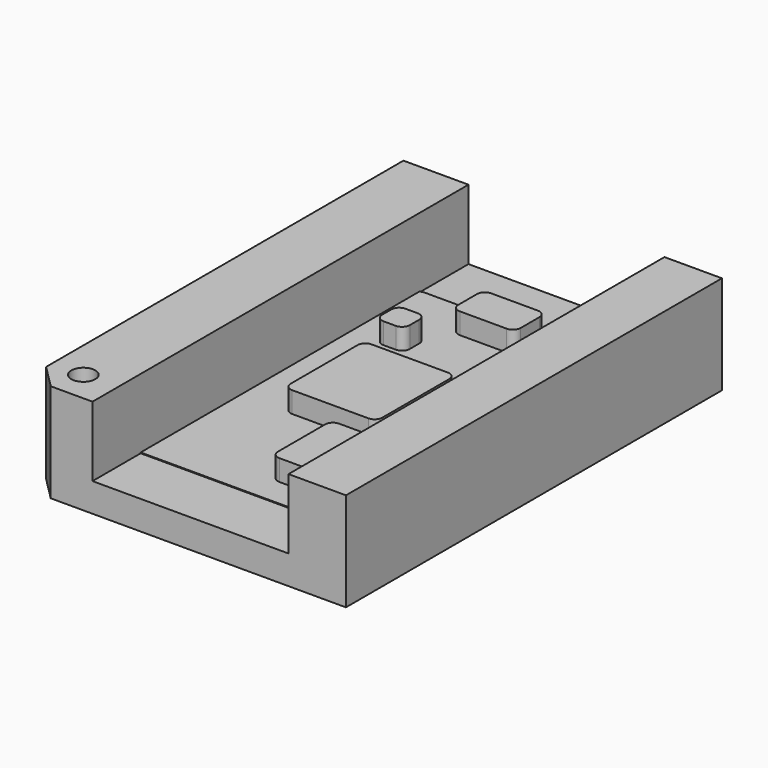
from build123d import *

# Parameters (mm, degrees)
F0_W      = 41
F0_H      = 60.5
F1_DEPTH  = 12.7
F2_R      = 1.54
F3_DEPTH  = 25
F4_W      = 25.2301925793
F4_H      = 60.5
F5_DEPTH  = 9
F6_W      = 30
F6_H      = 45
F7_DEPTH  = 3.8
F8_W      = 11.8106110021
F8_H      = 12.7719389275
F8_W_2    = 8.9266251307
F8_H_2    = 9.6132867038
F8_W_3    = 8.0407429487
F8_H_3    = 5.028893277
F8_W_4    = 3.5852673464
F8_H_4    = 3.5143401474
F9_DEPTH  = 2.7
F11_DEPTH = 25
F12_R     = 1
F13_R     = 1


with BuildPart() as f1:
    # F0 (on Top) → F1 (new body)
    with BuildSketch(Plane.XY):
        Rectangle(F0_W, F0_H)
    extrude(amount=F1_DEPTH)

    # F2 (on face) → F3 (cut)
    with BuildSketch(Plane.XY.offset(12.7)):
        Polygon((-17.5, -30.25), (-20.5, -27.25), (-20.5, -30.25), align=None)
        with Locations((-16.5, -26.25)):
            Circle(F2_R)
    extrude(amount=-F3_DEPTH, mode=Mode.SUBTRACT)

    # F4 (on face) → F5 (cut)
    with BuildSketch(Plane.XY.offset(12.7)):
        with Locations((0.4899087362, 0)):
            Rectangle(F4_W, F4_H)
    extrude(amount=-F5_DEPTH, mode=Mode.SUBTRACT)


with BuildPart() as f7:
    # F6 (on Top) → F7 (new body)
    with BuildSketch(Plane.XY):
        Rectangle(F6_W, F6_H)
    extrude(amount=F7_DEPTH)

    # F8 (on face) → F9 (join)
    with BuildSketch(Plane.XY.offset(3.8)):
        with Locations((-0.5493303761, -0.0686664134)):
            Rectangle(F8_W, F8_H)
        with Locations((6.2486376846, -14.0079334378)):
            Rectangle(F8_W_2, F8_H_2)
        with Locations((0, 19.9855533615)):
            Rectangle(F8_W_3, F8_H_3)
        with Locations((-6.8593251053, 12.7437841147)):
            Rectangle(F8_W_4, F8_H_4)
    extrude(amount=F9_DEPTH)

    # F10 (on face) → F11 (cut)
    with BuildSketch(Plane.XY.offset(3.8)):
        Polygon((-15, 22.5), (-15, 19.5), (-12, 22.5), align=None)
    extrude(amount=-F11_DEPTH, mode=Mode.SUBTRACT)

    # F12
    f12_edges = [f7.edges().sort_by_distance(p)[0] for p in [
        (15, 22.5, 1.9),
        (15, -22.5, 1.9),
        (-15, -22.5, 1.9),
        (-15, 19.5, 1.9),
        (-12, 22.5, 1.9),
    ]]
    fillet(f12_edges, radius=F12_R)

    # F13
    f13_edges = [f7.edges().sort_by_distance(p)[0] for p in [
        (5.355975, -6.454636, 5.15),
        (-6.454636, -6.454636, 5.15),
        (1.785325, -18.814577, 5.15),
        (10.71195, -18.814577, 5.15),
        (5.355975, 6.317303, 5.15),
        (-8.651959, 10.986614, 5.15),
        (-5.066691, 10.986614, 5.15),
        (-5.066691, 14.500954, 5.15),
        (-4.020371, 17.471107, 5.15),
        (4.020371, 17.471107, 5.15),
        (4.020371, 22.5, 5.15),
        (-6.454636, 6.317303, 5.15),
        (-8.651959, 14.500954, 5.15),
        (1.785325, -9.20129, 5.15),
        (-4.020371, 22.5, 5.15),
        (10.71195, -9.20129, 5.15),
    ]]
    fillet(f13_edges, radius=F13_R)


solid = Compound([f1.part, f7.part])
